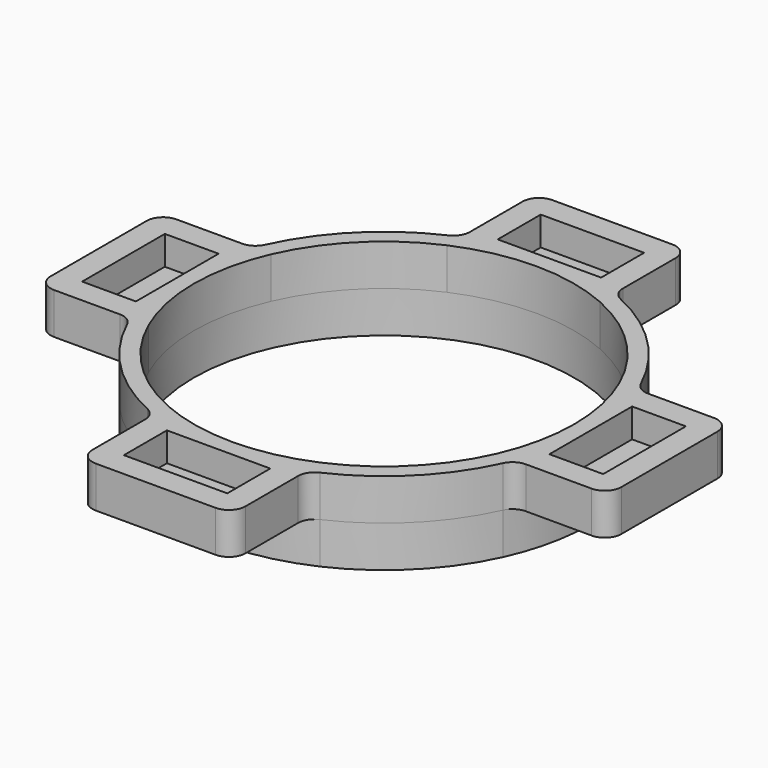
from build123d import *

# Parameters (mm, degrees)
F1_DEPTH = 5
F2_DEPTH = 3.5
F3_R     = 2
F4_R     = 23
F5_DEPTH = 5


# Not quite as in the source:
# - a feature names something its author has since deleted; it is built from what else it names


with BuildPart() as f1:
    # F0 (on Top) → F1 (new body)
    with BuildSketch(Plane.XY):
        with BuildLine():
            ThreePointArc((-25, 0), (-24.5524423049, 4.7093074719), (-23.2257938508, 9.25))
            Line((-23.2257938508, 9.25), (-34.5, 9.25))
            Line((-34.5, 9.25), (-34.5, -9.25))
            Line((-34.5, -9.25), (-23.2257938508, -9.25))
            ThreePointArc((-23.2257938508, -9.25), (-24.5524423049, -4.7093074719), (-25, 0))
        make_face()
        Polygon((-25, 6.25), (-25, 0), (-25, -6.25), (-31.5, -6.25), (-31.5, 6.25), align=None, mode=Mode.SUBTRACT)
        with BuildLine():
            Line((34.5, 9.25), (23.2257938508, 9.25))
            ThreePointArc((23.2257938508, 9.25), (24.5524423049, 4.7093074719), (25, 0))
            ThreePointArc((25, 0), (24.5524423049, -4.7093074719), (23.2257938508, -9.25))
            Line((23.2257938508, -9.25), (34.5, -9.25))
            Line((34.5, -9.25), (34.5, 9.25))
        make_face()
        Polygon((25, -6.25), (25, 0), (25, 6.25), (31.5, 6.25), (31.5, -6.25), align=None, mode=Mode.SUBTRACT)
        Polygon((-25, -6.25), (-25, 0), (-25, 6.25), (-31.5, 6.25), (-31.5, -6.25), align=None)
        Polygon((25, 6.25), (25, 0), (25, -6.25), (31.5, -6.25), (31.5, 6.25), align=None)
        with BuildLine():
            ThreePointArc((21.0579557412, 9.25), (22.5092534533, 4.7258342095), (23, 0))
            ThreePointArc((23, 0), (22.5092534533, -4.7258342095), (21.0579557412, -9.25))
            Line((21.0579557412, -9.25), (23.2257938508, -9.25))
            ThreePointArc((23.2257938508, -9.25), (24.5524423049, -4.7093074719), (25, 0))
            ThreePointArc((25, 0), (24.5524423049, 4.7093074719), (23.2257938508, 9.25))
            Line((23.2257938508, 9.25), (21.0579557412, 9.25))
        make_face()
        with BuildLine():
            ThreePointArc((9.25, 21.0579557412), (16.2634559673, 16.2634559673), (21.0579557412, 9.25))
            Line((21.0579557412, 9.25), (23.2257938508, 9.25))
            ThreePointArc((23.2257938508, 9.25), (17.6776695297, 17.6776695297), (9.25, 23.2257938508))
            Line((9.25, 23.2257938508), (9.25, 21.0579557412))
        make_face()
        with BuildLine():
            ThreePointArc((-21.0579557412, 9.25), (-16.2634559673, 16.2634559673), (-9.25, 21.0579557412))
            Line((-9.25, 21.0579557412), (-9.25, 23.2257938508))
            ThreePointArc((-9.25, 23.2257938508), (-17.6776695297, 17.6776695297), (-23.2257938508, 9.25))
            Line((-23.2257938508, 9.25), (-21.0579557412, 9.25))
        make_face()
        with BuildLine():
            Line((-9.25, -23.2257938508), (-9.25, -21.0579557412))
            ThreePointArc((-9.25, -21.0579557412), (-16.2634559673, -16.2634559673), (-21.0579557412, -9.25))
            Line((-21.0579557412, -9.25), (-23.2257938508, -9.25))
            ThreePointArc((-23.2257938508, -9.25), (-17.6776695297, -17.6776695297), (-9.25, -23.2257938508))
        make_face()
        with BuildLine():
            ThreePointArc((-21.0579557412, -9.25), (-23, 0), (-21.0579557412, 9.25))
            Line((-21.0579557412, 9.25), (-23.2257938508, 9.25))
            ThreePointArc((-23.2257938508, 9.25), (-24.5524423049, 4.7093074719), (-25, 0))
            ThreePointArc((-25, 0), (-24.5524423049, -4.7093074719), (-23.2257938508, -9.25))
            Line((-23.2257938508, -9.25), (-21.0579557412, -9.25))
        make_face()
        with BuildLine():
            ThreePointArc((-9.25, 21.0579557412), (0, 23), (9.25, 21.0579557412))
            Line((9.25, 21.0579557412), (9.25, 23.2257938508))
            ThreePointArc((9.25, 23.2257938508), (4.7093074719, 24.5524423049), (0, 25))
            ThreePointArc((0, 25), (-4.7093074719, 24.5524423049), (-9.25, 23.2257938508))
            Line((-9.25, 23.2257938508), (-9.25, 21.0579557412))
        make_face()
        with BuildLine():
            Line((23.2257938508, -9.25), (21.0579557412, -9.25))
            ThreePointArc((21.0579557412, -9.25), (16.2634559673, -16.2634559673), (9.25, -21.0579557412))
            Line((9.25, -21.0579557412), (9.25, -23.2257938508))
            ThreePointArc((9.25, -23.2257938508), (17.6776695297, -17.6776695297), (23.2257938508, -9.25))
        make_face()
        with BuildLine():
            Line((9.25, -23.2257938508), (9.25, -21.0579557412))
            ThreePointArc((9.25, -21.0579557412), (0, -23), (-9.25, -21.0579557412))
            Line((-9.25, -21.0579557412), (-9.25, -23.2257938508))
            ThreePointArc((-9.25, -23.2257938508), (-4.7093074719, -24.5524423049), (0, -25))
            ThreePointArc((0, -25), (4.7093074719, -24.5524423049), (9.25, -23.2257938508))
        make_face()
        with BuildLine():
            Line((9.25, -34.5), (9.25, -23.2257938508))
            ThreePointArc((9.25, -23.2257938508), (4.7093074719, -24.5524423049), (0, -25))
            ThreePointArc((0, -25), (-4.7093074719, -24.5524423049), (-9.25, -23.2257938508))
            Line((-9.25, -23.2257938508), (-9.25, -34.5))
            Line((-9.25, -34.5), (9.25, -34.5))
        make_face()
        Polygon((-6.25, -25), (0, -25), (6.25, -25), (6.25, -31.5), (-6.25, -31.5), align=None, mode=Mode.SUBTRACT)
        Polygon((6.25, -25), (0, -25), (-6.25, -25), (-6.25, -31.5), (6.25, -31.5), align=None)
        with BuildLine():
            ThreePointArc((0, 25), (4.7093074719, 24.5524423049), (9.25, 23.2257938508))
            Line((9.25, 23.2257938508), (9.25, 34.5))
            Line((9.25, 34.5), (-9.25, 34.5))
            Line((-9.25, 34.5), (-9.25, 23.2257938508))
            ThreePointArc((-9.25, 23.2257938508), (-4.7093074719, 24.5524423049), (0, 25))
        make_face()
        Polygon((6.25, 25), (0, 25), (-6.25, 25), (-6.25, 31.5), (6.25, 31.5), align=None, mode=Mode.SUBTRACT)
        Polygon((-6.25, 25), (0, 25), (6.25, 25), (6.25, 31.5), (-6.25, 31.5), align=None)
    extrude(amount=-F1_DEPTH)

    # F0 (on Top) → F2 (cut)
    with BuildSketch(Plane.XY):
        Polygon((-25, -6.25), (-25, 0), (-25, 6.25), (-31.5, 6.25), (-31.5, -6.25), align=None)
        Polygon((25, 6.25), (25, 0), (25, -6.25), (31.5, -6.25), (31.5, 6.25), align=None)
        Polygon((-6.25, 25), (0, 25), (6.25, 25), (6.25, 31.5), (-6.25, 31.5), align=None)
        Polygon((6.25, -25), (0, -25), (-6.25, -25), (-6.25, -31.5), (6.25, -31.5), align=None)
    extrude(amount=-F2_DEPTH, mode=Mode.SUBTRACT)

    # F3
    f3_edges = [f1.edges().sort_by_distance(p)[0] for p in [
        (-34.5, 9.25, -2.5),
        (-34.5, -9.25, -2.5),
        (34.5, 9.25, -2.5),
        (23.225794, -9.25, -2.5),
        (34.5, -9.25, -2.5),
        (-23.225794, -9.25, -2.5),
        (23.225794, 9.25, -2.5),
        (9.25, 34.5, -2.5),
        (9.25, 23.225794, -2.5),
        (9.25, -34.5, -2.5),
        (-9.25, -34.5, -2.5),
        (-9.25, -23.225794, -2.5),
        (9.25, -23.225794, -2.5),
        (-9.25, 34.5, -2.5),
        (-9.25, 23.225794, -2.5),
        (-23.225794, 9.25, -2.5),
    ]]
    fillet(f3_edges, radius=F3_R)

    # F4 (on face) → F5 (join)
    with BuildSketch(Plane(origin=(0, 0, -5), x_dir=(1, 0, 0), z_dir=(0, 0, -1))):
        with BuildLine():
            ThreePointArc((22.7264835722, -10.4166666667), (24.4250085906, -5.330943195), (25, 0))
            ThreePointArc((25, 0), (24.4250085906, 5.330943195), (22.7264835722, 10.4166666667))
            ThreePointArc((22.7264835722, 10.4166666667), (17.6776695297, 17.6776695297), (10.4166666667, 22.7264835722))
            ThreePointArc((10.4166666667, 22.7264835722), (0, 25), (-10.4166666667, 22.7264835722))
            ThreePointArc((-10.4166666667, 22.7264835722), (-17.6776695297, 17.6776695297), (-22.7264835722, 10.4166666667))
            ThreePointArc((-22.7264835722, 10.4166666667), (-25, 0), (-22.7264835722, -10.4166666667))
            ThreePointArc((-22.7264835722, -10.4166666667), (-17.6776695297, -17.6776695297), (-10.4166666667, -22.7264835722))
            ThreePointArc((-10.4166666667, -22.7264835722), (0, -25), (10.4166666667, -22.7264835722))
            ThreePointArc((10.4166666667, -22.7264835722), (17.6776695297, -17.6776695297), (22.7264835722, -10.4166666667))
        make_face()
        Circle(F4_R, mode=Mode.SUBTRACT)
    extrude(amount=F5_DEPTH)


solid = f1.part
